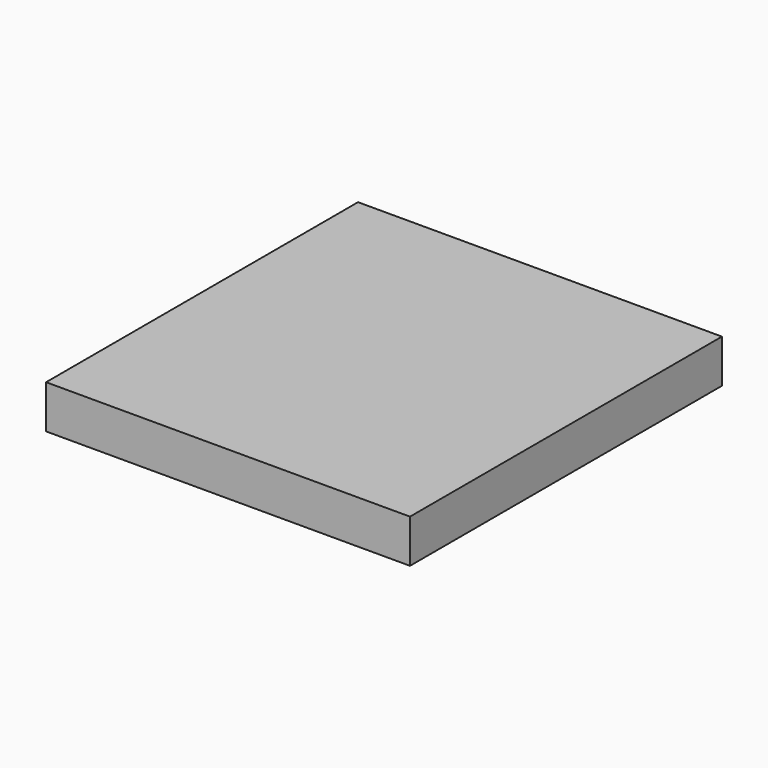
from build123d import *

# Parameters (mm, degrees)
F0_W     = 210
F0_H     = 225
F1_DEPTH = 12.5


# Not quite as in the source:
# - a feature names something its author has since deleted; it is built from what else it names


with BuildPart() as f1:
    # F0 (on Top) → F1 (new body, symmetric)
    with BuildSketch(Plane.XY):
        with Locations((9.306384975, 0.4089418799)):
            Rectangle(F0_W, F0_H)
    extrude(amount=F1_DEPTH, both=True)


solid = f1.part
